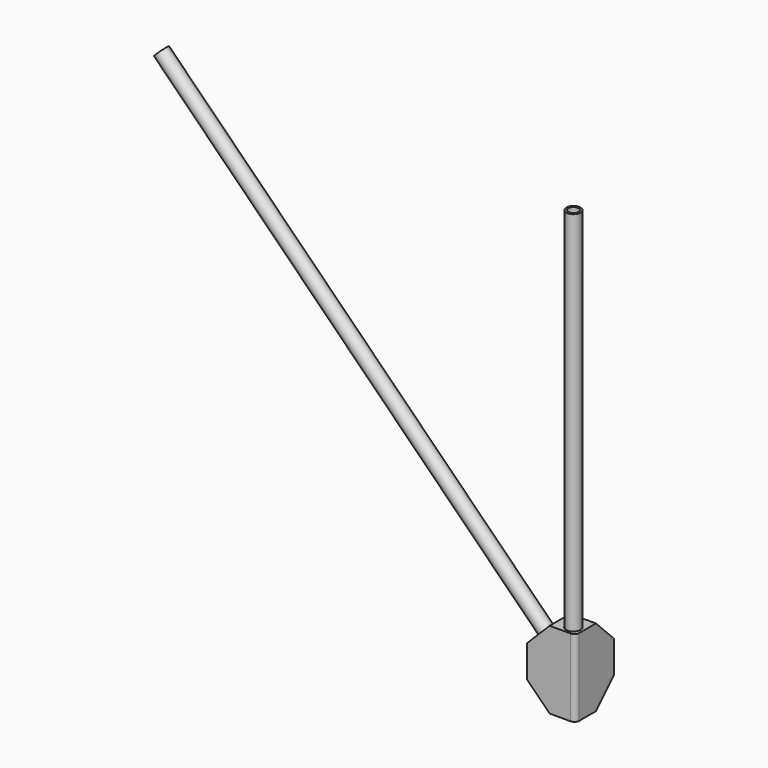
from build123d import *

# Parameters (mm, degrees)
F1_DEPTH  = 25.4
F2_SIZE   = 14.859
F3_R      = 3.175
F4_DEPTH  = 50.801
F5_R      = 3.175
F6_DEPTH  = 25.401
F7_R      = 3.175
F8_DEPTH  = 25.401
F9_R      = 3.175
F10_DEPTH = 25.4151248226
F11_R     = 3.175
F12_DEPTH = 25.4158319294
F13_R     = 3.175
F14_DEPTH = 25.4151248226
F15_R     = 3.175
F16_DEPTH = 25.4155629873
F17_R     = 3.175
F18_R     = 3.175
F19_R     = 4.7625
F20_DEPTH = 12.7
F21_R     = 4.7625
F22_DEPTH = 12.7
F23_R     = 4.7625
F24_DEPTH = 12.7
F25_R     = 4.7625
F26_DEPTH = 12.7
F27_R     = 4.7625
F28_DEPTH = 12.7
F29_R     = 4.7625
F30_DEPTH = 12.7
F31_R     = 4.7625
F32_DEPTH = 12.7
F33_R     = 4.7625
F36_DEPTH = 12.7
F37_R     = 4.6355
F37_R_2   = 3.3655
F38_DEPTH = 254
F39_R     = 4.6355
F39_R_2   = 3.3655
F40_DEPTH = 370.0574209815


# Not quite as in the source:
# - a variable given as a bare number and used for a length is read in inches; the dataset says mm whatever the document's units were


with BuildPart() as f1:
    # F0 (on Top) → F1 (new body, symmetric)
    with BuildSketch(Plane.XY):
        Polygon((-6.35, 25.4), (-6.35, 6.35), (-25.4, 6.35), (-25.4, -6.35), (6.35, -6.35), (6.35, 25.4), align=None)
    extrude(amount=F1_DEPTH, both=True)

    # F2
    f2_edges = [f1.edges().sort_by_distance(p)[0] for p in [
        (-25.4, 0, 25.4),
        (-25.4, 0, -25.4),
        (0, 25.4, -25.4),
        (0, 25.4, 25.4),
    ]]
    chamfer(f2_edges, length=F2_SIZE)

    # F3 (on face) → F4 (cut, through all)
    with BuildSketch(Plane.XY.offset(25.4)):
        Circle(F3_R)
    extrude(amount=-F4_DEPTH, mode=Mode.SUBTRACT)

    # F5 (on face) → F6 (cut, through all)
    with BuildSketch(Plane(origin=(-25.4, 0, 0), x_dir=(0, -1, 0), z_dir=(-1, 0, 0))):
        Circle(F5_R)
    extrude(amount=-F6_DEPTH, mode=Mode.SUBTRACT)

    # F7 (on face) → F8 (cut, through all)
    with BuildSketch(Plane(origin=(0, 25.4, 0), x_dir=(-1, 0, 0), z_dir=(0, 1, 0))):
        Circle(F7_R)
    extrude(amount=-F8_DEPTH, mode=Mode.SUBTRACT)

    # F9 (on face) → F10 (cut, through all)
    with BuildSketch(Plane(origin=(0, 17.9705, 17.9705), x_dir=(-1, 0, 0), z_dir=(0, 0.7071067812, 0.7071067812))):
        Circle(F9_R)
    extrude(amount=-F10_DEPTH, mode=Mode.SUBTRACT)

    # F11 (on face) → F12 (cut, through all)
    with BuildSketch(Plane(origin=(-17.9705, 0, 17.9705), x_dir=(0, -1, 0), z_dir=(-0.7071067812, 0, 0.7071067812))):
        Circle(F11_R)
    extrude(amount=-F12_DEPTH, mode=Mode.SUBTRACT)

    # F13 (on face) → F14 (cut, through all)
    with BuildSketch(Plane(origin=(0, 17.9705, -17.9705), x_dir=(-1, 0, 0), z_dir=(0, 0.7071067812, -0.7071067812))):
        Circle(F13_R)
    extrude(amount=-F14_DEPTH, mode=Mode.SUBTRACT)

    # F15 (on face) → F16 (cut, through all)
    with BuildSketch(Plane(origin=(-17.9705, 0, -17.9705), x_dir=(0, -1, 0), z_dir=(-0.7071067812, 0, -0.7071067812))):
        Circle(F15_R)
    extrude(amount=-F16_DEPTH, mode=Mode.SUBTRACT)

    # F17
    f17_edges = [f1.edges().sort_by_distance(p)[0] for p in [
        (-6.35, 6.35, 0),
    ]]
    fillet(f17_edges, radius=F17_R)

    # F18
    f18_edges = [f1.edges().sort_by_distance(p)[0] for p in [
        (6.35, -6.35, 0),
    ]]
    fillet(f18_edges, radius=F18_R)

    # F19 (on face) → F20 (cut)
    with BuildSketch(Plane(origin=(0, 0, -25.4), x_dir=(1, 0, 0), z_dir=(0, 0, -1))):
        Circle(F19_R)
    extrude(amount=-F20_DEPTH, mode=Mode.SUBTRACT)

    # F21 (on face) → F22 (cut)
    with BuildSketch(Plane.XY.offset(25.4)):
        Circle(F21_R)
    extrude(amount=-F22_DEPTH, mode=Mode.SUBTRACT)

    # F23 (on face) → F24 (cut)
    with BuildSketch(Plane(origin=(-25.4, 0, 0), x_dir=(0, -1, 0), z_dir=(-1, 0, 0))):
        Circle(F23_R)
    extrude(amount=-F24_DEPTH, mode=Mode.SUBTRACT)

    # F25 (on face) → F26 (cut)
    with BuildSketch(Plane(origin=(0, 25.4, 0), x_dir=(-1, 0, 0), z_dir=(0, 1, 0))):
        Circle(F25_R)
    extrude(amount=-F26_DEPTH, mode=Mode.SUBTRACT)

    # F27 (on face) → F28 (cut)
    with BuildSketch(Plane(origin=(-17.9705, 0, 17.9705), x_dir=(0, -1, 0), z_dir=(-0.7071067812, 0, 0.7071067812))):
        Circle(F27_R)
    extrude(amount=-F28_DEPTH, mode=Mode.SUBTRACT)

    # F29 (on face) → F30 (cut)
    with BuildSketch(Plane(origin=(0, 17.9705, 17.9705), x_dir=(-1, 0, 0), z_dir=(0, 0.7071067812, 0.7071067812))):
        Circle(F29_R)
    extrude(amount=-F30_DEPTH, mode=Mode.SUBTRACT)

    # F31 (on face) → F32 (cut)
    with BuildSketch(Plane(origin=(0, 17.9705, -17.9705), x_dir=(-1, 0, 0), z_dir=(0, 0.7071067812, -0.7071067812))):
        Circle(F31_R)
    extrude(amount=-F32_DEPTH, mode=Mode.SUBTRACT)

    # F33 (on face) → F36 (cut)
    with BuildSketch(Plane(origin=(-17.9705, 0, -17.9705), x_dir=(0, -1, 0), z_dir=(-0.7071067812, 0, -0.7071067812))):
        Circle(F33_R)
    extrude(amount=-F36_DEPTH, mode=Mode.SUBTRACT)


with BuildPart() as f38:
    # F37 (on face) → F38 (new body)
    with BuildSketch(Plane.XY.offset(12.7)):
        Circle(F37_R)
        Circle(F37_R_2, mode=Mode.SUBTRACT)
    extrude(amount=F38_DEPTH)


with BuildPart() as f40:
    # F39 (on face) → F40 (new body)
    with BuildSketch(Plane(origin=(-8.9902438789, 0, 8.9902438789), x_dir=(0, -1, 0), z_dir=(-0.7071067812, 0, 0.7071067812))):
        Circle(F39_R)
        Circle(F39_R_2, mode=Mode.SUBTRACT)
    extrude(amount=F40_DEPTH)


solid = Compound([f1.part, f38.part, f40.part])
